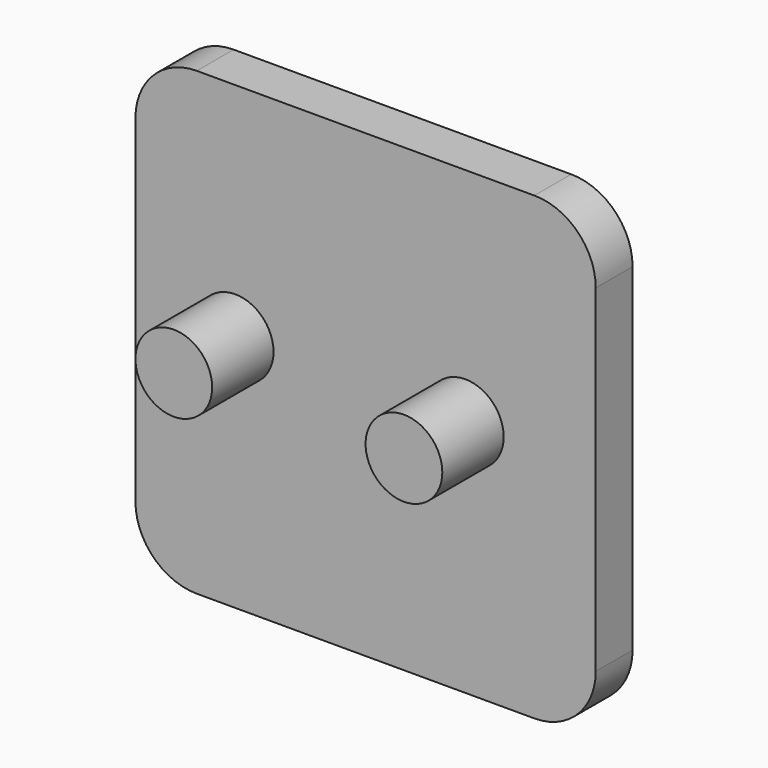
from build123d import *

# Parameters (mm, degrees)
F1_W           = 38.1
F1_H           = 38.1
F2_DEPTH       = 3.81
F3_R           = 3.175
F4_DEPTH       = 6.35
F5_R           = 5.08
F8_DEPTH       = 0.3175
F9_TEXT_SIZE   = 4.9309210024
F9_TEXT_SIZE_2 = 5.0353533071
F9_TEXT_SIZE_3 = 3.7948212897
F9_TEXT_SIZE_4 = 3.4233063666
F9_TEXT_SIZE_5 = 4.286538913
F9_TEXT_SIZE_6 = 3.7378385767
F9_TEXT_SIZE_7 = 4.2485771701
F9_TEXT_SIZE_8 = 4.0491771263
F10_DEPTH      = 0.3175
F11_W          = 23.3954964206
F11_H          = 0.4370380193
F12_DEPTH      = 0.3175


# Not quite as in the source:
# - Text() gives the source's letters only with a copy of the font that has no kerning and outlines rounded to 1/6400 em; it was checked with that copy


with BuildPart() as f2:
    # F1 (on offset) → F2 (new body)
    with BuildSketch(Plane.XZ.offset(25.4)):
        with Locations((-21.425308247, 18.5530144557)):
            Rectangle(F1_W, F1_H)
    extrude(amount=F2_DEPTH)

    # F3 (on face) → F4 (join)
    with BuildSketch(Plane.XZ.offset(29.21)):
        with Locations((-32.220308247, 19.1880144557)):
            Circle(F3_R)
        with Locations((-13.170308247, 19.1880144557)):
            Circle(F3_R)
    extrude(amount=F4_DEPTH)

    # F5
    f5_edges = [f2.edges().sort_by_distance(p)[0] for p in [
        (-40.475308, -27.305, 37.603014),
        (-2.375308, -27.305, 37.603014),
        (-40.475308, -27.305, -0.496986),
        (-2.375308, -27.305, -0.496986),
    ]]
    fillet(f5_edges, radius=F5_R)

    # F7 (on face) → F8 (cut)
    with BuildSketch(Plane(origin=(0, -25.4, 0), x_dir=(-1, 0, 0), z_dir=(0, 1, 0))):
        Polygon((12.6290200278, 34.7187258303), (3.9102202281, 34.7187258303), (6.485377904, 30.033910647), (6.8833935075, 5.9753647074), (6.922697669, 3.5995759973), (7.0077003911, 3.6009822506), (9.9715990946, 3.3956870902), (19.0850868821, 3.3956870902), (21.8502487987, 1.3529333519), (24.1223294288, 3.4225911368), (33.3103425801, 3.4225911368), (36.4377573133, 3.7207957357), (36.4377573133, 6.6668614745), (36.4377573133, 30.2996654063), (38.733985275, 34.526322037), (30.3983259946, 34.526322037), (30.0873341929, 34.526322037), (28.7930704653, 33.3972908556), (27.6523139328, 34.7049959274), (15.4967862216, 34.7049959274), (13.875534758, 33.2902558148), align=None)
    extrude(amount=-F8_DEPTH, mode=Mode.SUBTRACT)

    # F9 (on face) → F10 (join)
    with BuildSketch(Plane(origin=(0, -25.7175, 0), x_dir=(-1, 0, 0), z_dir=(0, 1, 0))):
        with Locations((8.5596432909, 26.6461465508)):
            Text('NEW YORK', F9_TEXT_SIZE, font='Open Sans', text_align=(TextAlign.LEFT, TextAlign.BOTTOM))
        with Locations((12.3642468825, 20.8774860948)):
            Text('R', F9_TEXT_SIZE_2, font='Open Sans', text_align=(TextAlign.LEFT, TextAlign.BOTTOM))
        with Locations((15.7174774754, 18.1452147663)):
            Text('A', F9_TEXT_SIZE_3, font='Open Sans', text_align=(TextAlign.LEFT, TextAlign.BOTTOM))
        with Locations((18.3649582658, 15.6804341823)):
            Text('N', F9_TEXT_SIZE_4, font='Open Sans', text_align=(TextAlign.LEFT, TextAlign.BOTTOM))
        with Locations((20.8318784163, 12.5941261649)):
            Text('G', F9_TEXT_SIZE_5, font='Open Sans', text_align=(TextAlign.LEFT, TextAlign.BOTTOM))
        with Locations((23.9168468902, 9.9028823897)):
            Text('E', F9_TEXT_SIZE_6, font='Open Sans', text_align=(TextAlign.LEFT, TextAlign.BOTTOM))
        with Locations((26.0135407168, 6.8439068273)):
            Text('R', F9_TEXT_SIZE_7, font='Open Sans', text_align=(TextAlign.LEFT, TextAlign.BOTTOM))
        with Locations((28.842827576, 3.9284992963)):
            Text('S', F9_TEXT_SIZE_8, font='Open Sans', text_align=(TextAlign.LEFT, TextAlign.BOTTOM))
    extrude(amount=F10_DEPTH)

    # F11 (on face) → F12 (join)
    with BuildSketch(Plane(origin=(0, -25.7175, 0), x_dir=(-1, 0, 0), z_dir=(0, 1, 0))):
        Polygon((33.4452651441, 31.8002551794), (9.1137969866, 31.8002551794), (9.1137969866, 31.0502536595), (33.4361046553, 31.0502536595), align=None)
        with Locations((21.4764908887, 25.272234343)):
            Rectangle(F11_W, F11_H)
        Polygon((33.1404767931, 6.2463656068), (17.2851830721, 24.3508461863), (16.5846580667, 23.7373500039), (32.3622695158, 5.7215714823), align=None)
        Polygon((25.6654638797, 4.1531343013), (11.0986828804, 21.7329673469), (10.5251273047, 21.2577149119), (24.9211379517, 3.8839750506), align=None)
    extrude(amount=F12_DEPTH)


solid = f2.part
